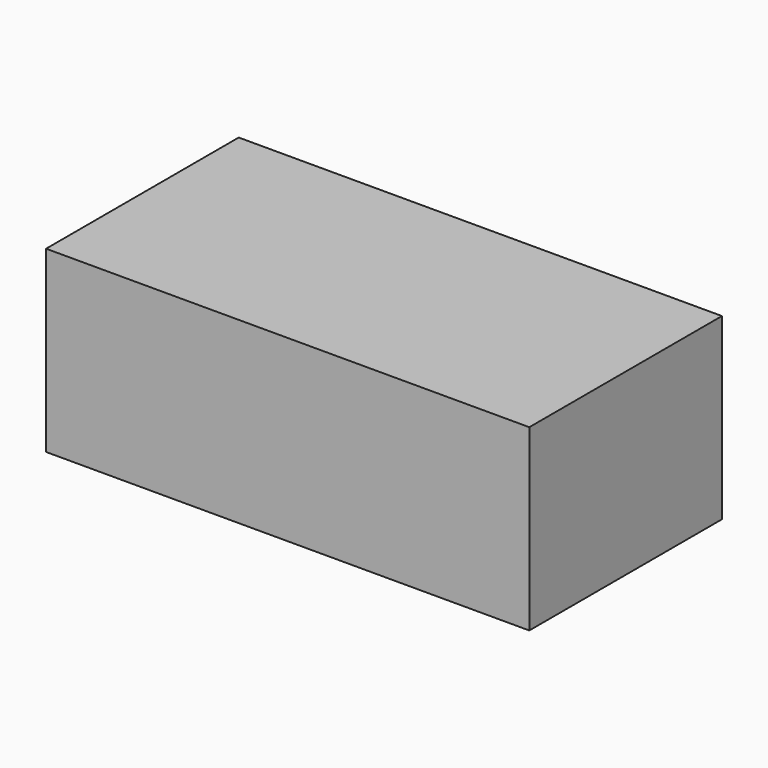
from build123d import *

# Parameters (mm, degrees)
F1_E1_W  = 64.3864218146
F1_E1_H  = 44.7370987386
F2_DEPTH = 33.2531612366


# Not quite as in the source:
# - a feature of the source that left no trace in its solid (it failed there, or was rolled back) is left out
# - a pattern or mirror of a feature is missing from the dataset's text; its kind, count and spacing are read off the source's solid


with BuildPart() as f2:
    # F1_E1 (on explicit) → F2 (new body)
    with BuildSketch(Plane(origin=(-13.9645393938, 0, -22.8319708258), x_dir=(1, 0, 0), z_dir=(0, 0, -1))):
        with Locations((32.1932109073, 22.3685493693)):
            Rectangle(F1_E1_W, F1_E1_H)
    extrude(amount=F2_DEPTH)

    # F2_copies: F2 across plane


with BuildPart() as f2_1:
    add(f2.part)
    add(f2.part.mirror(Plane(origin=(30.928672, 0, 0), x_dir=(0, 0, 1), z_dir=(1, 0, 0))))


solid = f2_1.part
